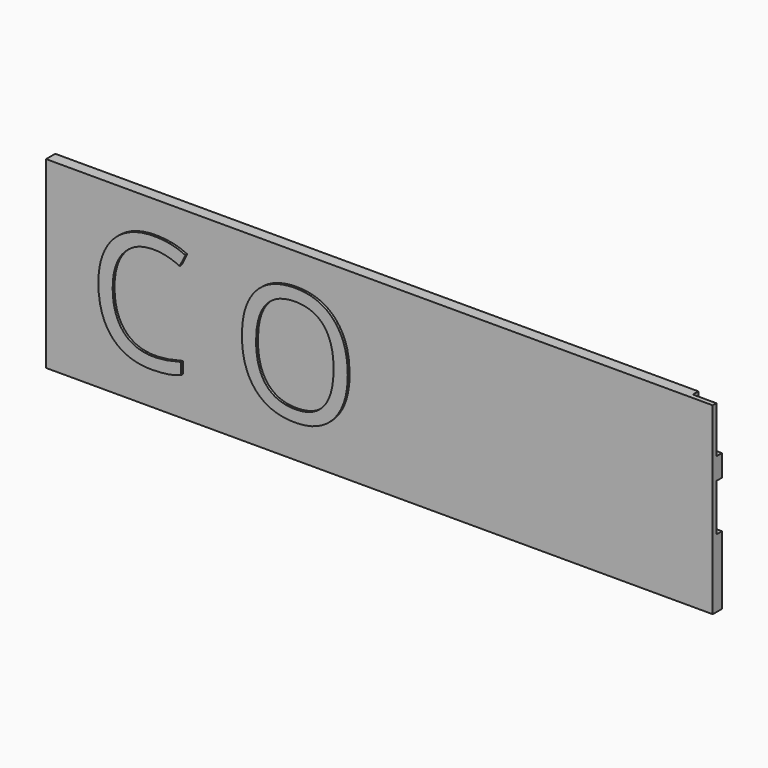
from build123d import *

# Parameters (mm, degrees)
F1_TEXT_SIZE = 44.5169422569
F2_DEPTH     = 0.635
F0_W         = 184.15
F0_H         = 50.8
F3_DEPTH     = 3.175
F4_W         = 184.15
F4_H         = 13.0136748776
F5_DEPTH     = 1.905
F7_W         = 19.05
F7_H         = 39.891424209
F8_DEPTH     = 13.208
F9_W         = 6.604
F9_H         = 12.954
F10_DEPTH    = 1.905


# Not quite as in the source:
# - Text() gives the source's letters only with a copy of the font that has no kerning and outlines rounded to 1/6400 em; it was checked with that copy


with BuildPart() as f2:
    # F1 (on face) → F2 (new body, symmetric)
    with BuildSketch(Plane.XZ):
        with Locations((-79.8400901084, -15.4407267692)):
            Text('C O', F1_TEXT_SIZE, font='Open Sans', text_align=(TextAlign.LEFT, TextAlign.BOTTOM))
    extrude(amount=F2_DEPTH, both=True)


with BuildPart() as f3:
    # F0 (on Front) → F3 (new body)
    with BuildSketch(Plane.XZ):
        Rectangle(F0_W, F0_H)
    extrude(amount=-F3_DEPTH)

    # F4 (on face) → F5 (cut)
    with BuildSketch(Plane(origin=(0, 3.175, 0), x_dir=(-1, 0, 0), z_dir=(0, 1, 0))):
        Rectangle(F4_W, F4_H)
    extrude(amount=-F5_DEPTH, mode=Mode.SUBTRACT)

    # F7 (on face) → F8 (cut)
    with BuildSketch(Plane(origin=(0, 1.27, 0), x_dir=(-1, 0, 0), z_dir=(0, 1, 0))):
        with Locations((82.5785435736, -0.2066679299)):
            Rectangle(F7_W, F7_H)
    extrude(amount=F8_DEPTH, mode=Mode.SUBTRACT)

    # F9 (on face) → F10 (cut)
    with BuildSketch(Plane(origin=(0, 3.175, 0), x_dir=(-1, 0, 0), z_dir=(0, 1, 0))):
        with Locations((-88.8686706285, 18.9704492633)):
            Rectangle(F9_W, F9_H)
    extrude(amount=-F10_DEPTH, mode=Mode.SUBTRACT)


solid = Compound([f2.part, f3.part])
